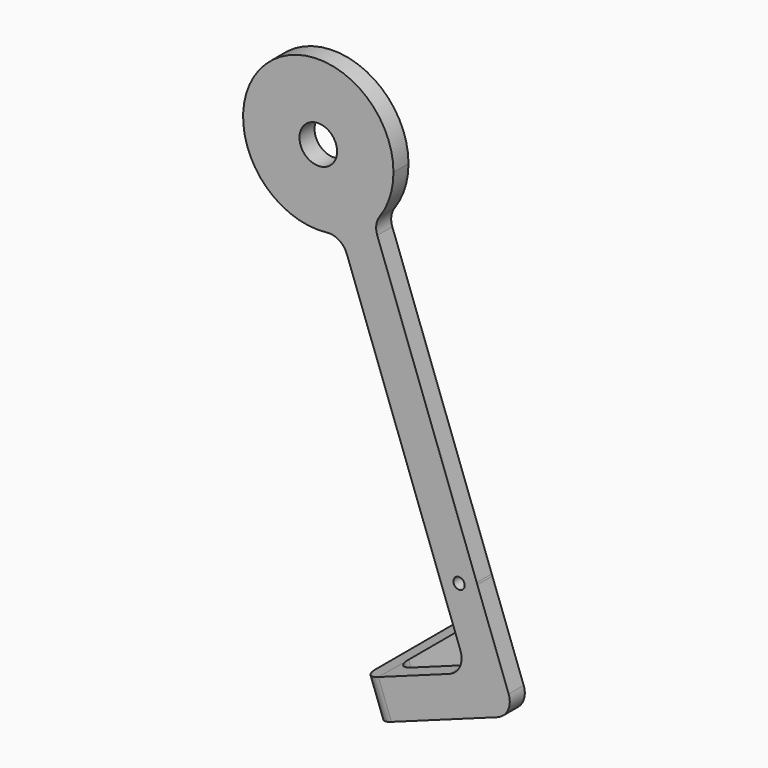
from build123d import *

# Parameters (mm, degrees)
F0_R     = 5
F0_R_2   = 1.5
F1_DEPTH = 5
F2_DEPTH = 35
F3_R     = 4.99999


# Not quite as in the source:
# - a fillet or chamfer is up to 0.001 mm smaller than in the source, because OpenCascade refuses the exact size


with BuildPart() as f1:
    # F0 (on Front) → F1 (new body)
    with BuildSketch(Plane.XZ):
        with BuildLine():
            ThreePointArc((14.7291057085, 20.287369527), (18.6357467541, 26.5570015397), (20, 33.8170940264))
            ThreePointArc((20, 33.8170940264), (-16.154238453, 45.6086409989), (6.0959419995, 14.7687478741))
            ThreePointArc((6.0959419995, 14.7687478741), (10.7719287617, 16.9658166044), (14.7291057085, 20.287369527))
        make_face()
        with Locations((0, 33.8170940264)):
            Circle(F0_R, mode=Mode.SUBTRACT)
        with BuildLine():
            ThreePointArc((14.7291057085, 20.287369527), (10.7719287617, 16.9658166044), (6.0959419995, 14.7687478741))
            Line((6.0959419995, 14.7687478741), (32.0687023036, -56.5908245822))
            Line((32.0687023036, -56.5908245822), (32.4609528428, -56.4480570615))
            ThreePointArc((32.4609528428, -56.4480570615), (36.7371185385, -51.8113638587), (42.1496687351, -55.0500082175))
            Line((42.1496687351, -55.0500082175), (14.7291057085, 20.287369527))
        make_face()
        with BuildLine():
            Line((32.4609528428, -56.4480570615), (32.0687023036, -56.5908245822))
            Line((32.0687023036, -56.5908245822), (32.5817325186, -58.0003635134))
            Line((32.5817325186, -58.0003635134), (32.7527425708, -58.4702097705))
            ThreePointArc((32.7527425708, -58.4702097705), (32.5024604285, -57.4741961437), (32.4609528428, -56.4480570615))
        make_face()
        with BuildLine():
            ThreePointArc((33.8290334161, -60.2068275447), (33.2012405538, -59.3940787929), (32.7527425708, -58.4702097705))
            Line((32.7527425708, -58.4702097705), (33.4367828769, -60.3495950653))
            Line((33.4367828769, -60.3495950653), (33.8290334161, -60.2068275447))
        make_face()
        with BuildLine():
            ThreePointArc((42.4512056942, -56.7601091071), (42.3752444432, -55.8918681281), (42.1496687351, -55.0500082175))
            ThreePointArc((42.1496687351, -55.0500082175), (36.7371185385, -51.8113638587), (32.4609528428, -56.4480570615))
            ThreePointArc((32.4609528428, -56.4480570615), (32.5024604285, -57.4741961437), (32.7527425708, -58.4702097705))
            ThreePointArc((32.7527425708, -58.4702097705), (33.2012405538, -59.3940787929), (33.8290334161, -60.2068275447))
            ThreePointArc((33.8290334161, -60.2068275447), (39.3071607865, -61.4028917528), (42.4512056942, -56.7601091071))
        make_face()
        with Locations((37.4512056942, -56.7601091071)):
            Circle(F0_R_2, mode=Mode.SUBTRACT)
        with BuildLine():
            Line((42.3206788698, -55.5198547009), (42.1496687351, -55.0500082175))
            ThreePointArc((42.1496687351, -55.0500082175), (42.3752444432, -55.8918681281), (42.4512056942, -56.7601091071))
            ThreePointArc((42.4512056942, -56.7601091071), (39.3071607865, -61.4028917528), (33.8290334161, -60.2068275447))
            Line((33.8290334161, -60.2068275447), (33.4367828769, -60.3495950653))
            Line((33.4367828769, -60.3495950653), (33.6077929485, -60.8194413757))
            Line((33.6077929485, -60.8194413757), (39.5341938332, -77.1020939848))
            Line((39.5341938332, -77.1020939848), (42.9543952664, -86.4990201927))
            Line((42.9543952664, -86.4990201927), (52.3513214743, -83.0788187594))
            Line((52.3513214743, -83.0788187594), (42.3206788698, -55.5198547009))
        make_face()
        Polygon((19.4620797468, -95.0495237758), (42.9543952664, -86.4990201927), (39.5341938332, -77.1020939848), (16.0418783135, -85.652597568), align=None)
        Polygon((14.7636166428, -96.7596244924), (19.4620797468, -95.0495237758), (16.0418783135, -85.652597568), (11.3434152096, -87.3626982846), align=None)
    extrude(amount=F1_DEPTH)

    # F0 (on Front) → F2 (join)
    with BuildSketch(Plane.XZ):
        Polygon((14.7636166428, -96.7596244924), (19.4620797468, -95.0495237758), (16.0418783135, -85.652597568), (11.3434152096, -87.3626982846), align=None)
    extrude(amount=-F2_DEPTH)

    # F3 (radius 5 in the source; OpenCascade refuses exactly that, so slightly less here)
    f3_edges = [f1.edges().sort_by_distance(p)[0] for p in [
        (6.095942, -2.5, 14.768748),
        (14.729106, -2.5, 20.28737),
        (52.351321, -2.5, -83.078819),
        (17.751979, 0, -90.351061),
        (13.053516, -5, -92.061161),
        (39.534194, -2.5, -77.102094),
        (17.751979, 35, -90.351061),
    ]]
    fillet(f3_edges, radius=F3_R)


solid = f1.part
